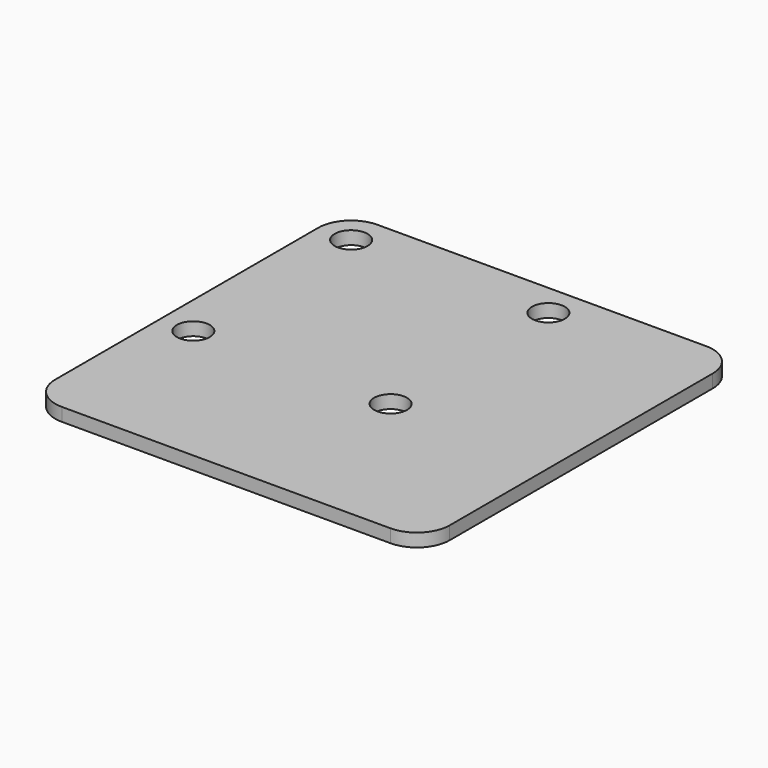
from build123d import *

# Parameters (mm, degrees)
F0_R     = 2.5
F1_DEPTH = 2


# Not quite as in the source:
# - a feature names something its author has since deleted; it is built from what else it names


with BuildPart() as f1:
    # F0 (on Top) → F1 (new body)
    with BuildSketch(Plane.XY):
        with BuildLine():
            ThreePointArc((40, 15), (38.5355339059, 18.5355339059), (35, 20))
            Line((35, 20), (-15, 20))
            ThreePointArc((-15, 20), (-18.5355339059, 18.5355339059), (-20, 15))
            Line((-20, 15), (-20, -35))
            ThreePointArc((-20, -35), (-18.5355339059, -38.5355339059), (-15, -40))
            Line((-15, -40), (35, -40))
            ThreePointArc((35, -40), (38.5355339059, -38.5355339059), (40, -35))
            Line((40, -35), (40, 15))
        make_face()
        with Locations((-15, -15)):
            Circle(F0_R, mode=Mode.SUBTRACT)
        with Locations((15, -15)):
            Circle(F0_R, mode=Mode.SUBTRACT)
        with Locations((-15, 15)):
            Circle(F0_R, mode=Mode.SUBTRACT)
        with Locations((15, 15)):
            Circle(F0_R, mode=Mode.SUBTRACT)
    extrude(amount=F1_DEPTH)


solid = f1.part
